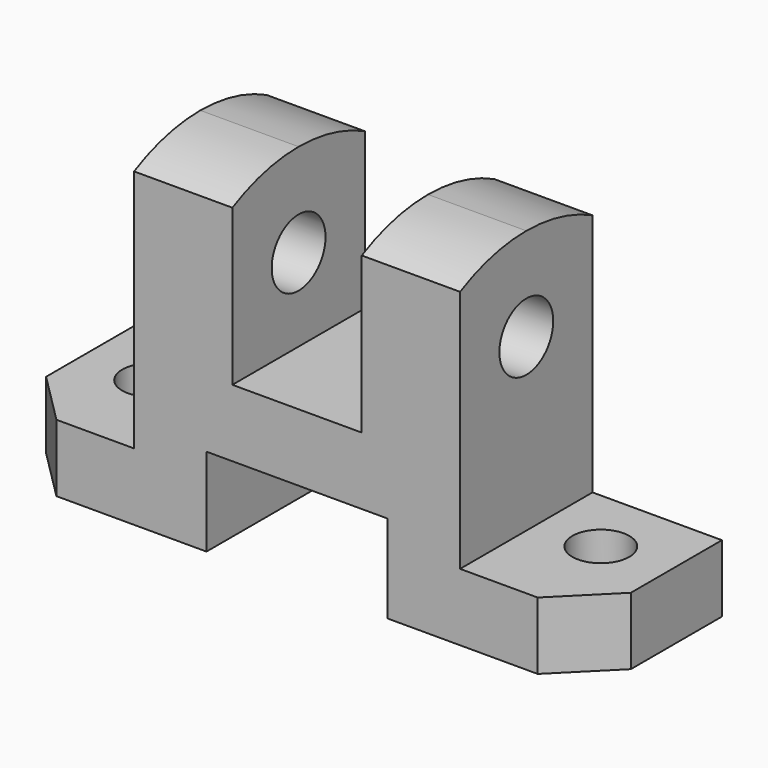
from build123d import *

# Parameters (mm, degrees)
F1_DEPTH = 32
F3_R     = 5.5
F2_R     = 5.5
F4_DEPTH = 13.001
F5_R     = 6.5
F6_DEPTH = 88.001


with BuildPart() as f1:
    # F0 (on Front) → F1 (new body)
    with BuildSketch(Plane.XZ):
        Polygon((-56.5, 13), (-56.5, 0), (-17.5, 0), (-17.5, 17), (17.5, 17), (17.5, 0), (56.5, 0), (56.5, 13), (31.5, 13), (31.5, 64), (12.5, 64), (12.5, 30), (-12.5, 30), (-12.5, 64), (-31.5, 64), (-31.5, 13), align=None)
    extrude(amount=F1_DEPTH)

    # F3 (on face) + F2 (on face) → F4 (cut, through all)
    with BuildSketch(Plane.XY.offset(13)):
        with Locations((-43.5, -13)):
            Circle(F3_R)
        Polygon((-46.5, -32), (-56.5, -22), (-56.5, -32), align=None)
    with BuildSketch(Plane.XY.offset(13)):
        with Locations((43.5, -13)):
            Circle(F2_R)
        Polygon((56.5, -22), (46.5, -32), (56.5, -32), align=None)
    extrude(amount=-F4_DEPTH, mode=Mode.SUBTRACT)

    # F5 (on face) → F6 (cut, through all)
    with BuildSketch(Plane.YZ.offset(31.5)):
        with Locations((-16, 46)):
            Circle(F5_R)
        with BuildLine():
            Line((-32, 64), (-32, 60.1287648325))
            ThreePointArc((-32, 60.1287648325), (-24.2308332161, 63.0184271325), (-16, 64))
            Line((-16, 64), (-32, 64))
        make_face()
        with BuildLine():
            Line((0, 64), (-16, 64))
            ThreePointArc((-16, 64), (-7.769166784, 63.0184271325), (0, 60.1287648325))
            Line((0, 60.1287648325), (0, 64))
        make_face()
    extrude(amount=-F6_DEPTH, mode=Mode.SUBTRACT)


solid = f1.part
